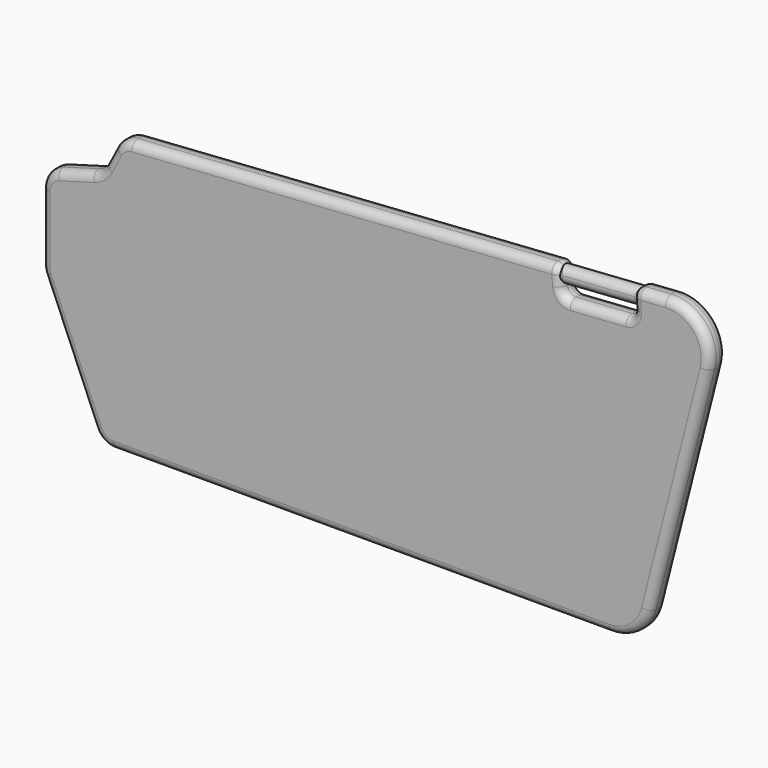
from build123d import *

# Parameters (mm, degrees)
F1_DEPTH      = 6.35
F2_R          = 12.7
F3_R          = 5.08
F5_DEPTH      = 50.8
F6_DEPTH      = 25.4
F7_T3_DEPTH   = 256.4039375074
F7_T6_DEPTH   = 256.4039375074
F7_T9_DEPTH   = 15.155251048
F7_T12_ANGLE  = 90
F7_S13_R      = 4.7625
F7_T14_DEPTH  = 6
F7_T17_ANGLE  = 108.2015581713
F7_T20_DEPTH  = 144.8369323212
F7_T23_ANGLE  = 90
F7_T26_ANGLE  = 75.7163995102
F7_T29_DEPTH  = 33.9682692967
F7_T32_DEPTH  = 302.1105912621
F7_T35_ANGLE  = 90
F7_T38_ANGLE  = 66.9516737984
F7_T41_DEPTH  = 78.7235310431
F7_T44_ANGLE  = 90
F7_S45_R      = 4.7625
F7_T46_DEPTH  = 6
F7_T49_ANGLE  = 23.0483262016
F7_T52_DEPTH  = 41.4021335168
F7_T55_ANGLE  = 58.5622729238
F7_T58_ANGLE  = 74.157776544
F7_T61_DEPTH  = 12.2118489341
F7_T64_DEPTH  = 22.3254991639
F7_T67_ANGLE  = 46.6380071493
F7_T70_DEPTH  = 15.155251048
F7_T73_ANGLE  = 90
F7_S74_R      = 4.7625
F7_T75_DEPTH  = 6
F7_T78_ANGLE  = 108.2015581713
F7_T81_DEPTH  = 144.8369323212
F7_T84_ANGLE  = 90
F7_T87_ANGLE  = 75.7163995102
F7_T90_DEPTH  = 33.9682692967
F7_T93_DEPTH  = 302.1105912621
F7_T96_ANGLE  = 90
F7_T99_ANGLE  = 66.9516737984
F7_T102_DEPTH = 78.7235310431
F7_T105_ANGLE = 90
F7_S106_R     = 4.7625
F7_T107_DEPTH = 6
F7_T110_ANGLE = 23.0483262016
F7_T113_DEPTH = 41.4021335168
F7_T116_ANGLE = 58.5622729238
F7_T119_ANGLE = 74.157776544
F7_T122_DEPTH = 12.2118489341
F7_T125_DEPTH = 22.3254991639
F7_T128_ANGLE = 46.6380071493
F7_T131_DEPTH = 6.35
F7_S132_R     = 4.7625
F7_T133_DEPTH = 7
F7_T136_DEPTH = 6.35
F7_S137_R     = 4.7625
F7_T138_DEPTH = 7
F7_T141_DEPTH = 6.35
F7_S142_R     = 4.7625
F7_T143_DEPTH = 7
F7_T146_DEPTH = 6.35
F7_S147_R     = 4.7625
F7_T148_DEPTH = 7


# Not quite as in the source:
# - a fillet or chamfer that OpenCascade refuses, or shapes differently, is made with other operations: its cross-section is extruded or revolved along the edge and cut away or added
# - a feature names something its author has since deleted; it is built from what else it names


with BuildPart() as f1:
    # F0 (on Front) → F1 (new body, symmetric)
    with BuildSketch(Plane.XZ):
        with BuildLine():
            Line((-207.3190157797, -14.1988740305), (-172.196418047, -96.7488740305))
            Line((-172.196418047, -96.7488740305), (138.3124196887, -96.7488740305))
            ThreePointArc((138.3124196887, -96.7488740305), (153.9006374043, -91.402987535), (162.9272139723, -77.6156038299))
            Line((162.9272139723, -77.6156038299), (198.6616202648, 62.7438959238))
            ThreePointArc((198.6616202648, 62.7438959238), (193.5563518445, 85.2752622268), (172.3112952336, 94.3512636991))
            Line((172.3112952336, 94.3512636991), (152.1233357391, 92.9686298258))
            Line((152.1233357391, 92.9686298258), (153.2514307251, 76.4972151415))
            Line((153.2514307251, 76.4972151415), (109.2262930579, 73.4820195428))
            Line((109.2262930579, 73.4820195428), (108.0981980719, 89.9534342271))
            Line((108.0981980719, 89.9534342271), (-159.8793958766, 71.6001727804))
            Line((-159.8793958766, 71.6001727804), (-171.3419263278, 49.5993942022))
            Line((-171.3419263278, 49.5993942022), (-207.3190157797, 39.3902622163))
            Line((-207.3190157797, 39.3902622163), (-207.3190157797, -14.1988740305))
        make_face()
    extrude(amount=F1_DEPTH, both=True)

    # F2
    f2_edges = [f1.edges().sort_by_distance(p)[0] for p in [
        (-171.341926, 0, 49.599394),
        (-207.319016, 0, 39.390262),
        (-159.879396, 0, 71.600173),
        (-207.319016, 0, -14.198874),
        (-172.196418, 0, -96.748874),
    ]]
    fillet(f2_edges, radius=F2_R)

    # F3
    f3_edges = [f1.edges().sort_by_distance(p)[0] for p in [
        (109.226293, 0, 73.48202),
        (153.251431, 0, 76.497215),
        (108.098198, 0, 89.953434),
        (152.123336, 0, 92.96863),
    ]]
    fillet(f3_edges, radius=F3_R)

    # F4 (on face) → F5 (join)
    with BuildSketch(Plane(origin=(113.7254907181, 0, 7.7888364977), x_dir=(0, 1, 0), z_dir=(0.9976629124, 0, 0.0683279822))):
        with BuildLine():
            Line((-4.686375775, 77.2770734216), (4.686375775, 77.2770734216))
            ThreePointArc((4.686375775, 77.2770734216), (0, 81.1914647341), (-4.686375775, 77.2770734216))
        make_face()
        with BuildLine():
            ThreePointArc((-4.686375775, 77.2770734216), (-0.4257590996, 71.6855339673), (4.7625, 76.4289647341))
            ThreePointArc((4.7625, 76.4289647341), (4.7434307668, 76.8547238336), (4.686375775, 77.2770734216))
            Line((4.686375775, 77.2770734216), (-4.686375775, 77.2770734216))
        make_face()
    extrude(amount=F5_DEPTH)

    # F6 (add): a face of the model
    f6_faces = [f1.faces().sort_by_distance(p)[0] for p in [
        (108.3333406106, 0, 86.5200972184),
    ]]
    extrude(f6_faces, amount=F6_DEPTH)

    # F7: fillet of radius 5.08 on 40 edges, made by hand


with BuildPart() as f7_tool1:
    # F7_s2 → F7_t3 (new body)
    with BuildSketch(Plane(origin=(108.657363123, 0, 7.4417303481), x_dir=(0, 1, 0), z_dir=(-0.9976629124, 0, -0.0683279822))):
        with BuildLine():
            ThreePointArc((-1.27, -82.3570734216), (-4.8621024484, -80.86917587), (-6.35, -77.2770734216))
            Line((-6.35, -77.2770734216), (-6.35, -82.3570734216))
            Line((-6.35, -82.3570734216), (-1.27, -82.3570734216))
        make_face()
    extrude(amount=F7_T3_DEPTH)


with BuildPart() as f7_tool4:
    # F7_s5 → F7_t6 (new body)
    with BuildSketch(Plane(origin=(108.657363123, 0, 7.4417303481), x_dir=(0, 1, 0), z_dir=(-0.9976629124, 0, -0.0683279822))):
        with BuildLine():
            ThreePointArc((6.35, -77.2770734216), (4.8621024484, -80.86917587), (1.27, -82.3570734216))
            Line((1.27, -82.3570734216), (6.35, -82.3570734216))
            Line((6.35, -82.3570734216), (6.35, -77.2770734216))
        make_face()
    extrude(amount=F7_T6_DEPTH)


with BuildPart() as f7_tool7:
    # F7_s8 → F7_t9 (new body)
    with BuildSketch(Plane(origin=(177.9385878798, 0, 12.1866659697), x_dir=(0, 1, 0), z_dir=(-0.9976629124, 0, -0.0683279822))):
        with BuildLine():
            ThreePointArc((6.35, -77.2770734216), (4.8621024484, -80.86917587), (1.27, -82.3570734216))
            Line((1.27, -82.3570734216), (6.35, -82.3570734216))
            Line((6.35, -82.3570734216), (6.35, -77.2770734216))
        make_face()
    extrude(amount=F7_T9_DEPTH)


with BuildPart() as f7_tool10:
    # F7_s11 → F7_t12 (revolve)
    with BuildSketch(Plane(origin=(162.8187559806, 0, 11.1511382459), x_dir=(0, 1, 0), z_dir=(0.9976629124, 0, 0.0683279822))):
        with BuildLine():
            ThreePointArc((6.35, 77.2770734216), (4.8621024484, 80.86917587), (1.27, 82.3570734216))
            Line((1.27, 82.3570734216), (6.35, 82.3570734216))
            Line((6.35, 82.3570734216), (6.35, 77.2770734216))
        make_face()
    revolve(axis=Axis((157.5385694838, 6.35, 88.2476083802), (0, -1, 0)), revolution_arc=F7_T12_ANGLE)

    # F7_s13 → F7_t14 (cut, symmetric)
    with BuildSketch(Plane(origin=(160.4241963196, 0, 10.9871395367), x_dir=(0, 1, 0), z_dir=(-0.9976629124, 0, -0.0683279822))):
        with Locations((0, -76.4289647341)):
            Circle(F7_S13_R)
    extrude(amount=F7_T14_DEPTH, both=True, mode=Mode.SUBTRACT)


with BuildPart() as f7_tool15:
    # F7_s16 → F7_t17 (revolve)
    with BuildSketch(Plane(origin=(27.0945707988, 0, 106.4234948309), x_dir=(0, 1, 0), z_dir=(-0.2467216456, 0, -0.9690863891))):
        with BuildLine():
            ThreePointArc((6.35, 171.9599949818), (4.8621024484, 175.5520974303), (1.27, 177.0399949818))
            Line((1.27, 177.0399949818), (6.35, 177.0399949818))
            Line((6.35, 177.0399949818), (6.35, 171.9599949818))
        make_face()
    revolve(axis=Axis((174.0468259813, 6.35, 69.0106257232), (0, -1, 0)), revolution_arc=F7_T17_ANGLE)


with BuildPart() as f7_tool18:
    # F7_s19 → F7_t20 (new body)
    with BuildSketch(Plane(origin=(-8.6398354938, 0, -33.9360049229), x_dir=(0, 1, 0), z_dir=(0.2467216456, 0, 0.9690863891))):
        with BuildLine():
            ThreePointArc((6.35, -171.9599949818), (4.8621024484, -175.5520974303), (1.27, -177.0399949818))
            Line((1.27, -177.0399949818), (6.35, -177.0399949818))
            Line((6.35, -177.0399949818), (6.35, -171.9599949818))
        make_face()
    extrude(amount=F7_T20_DEPTH)


with BuildPart() as f7_tool21:
    # F7_s22 → F7_t23 (revolve)
    with BuildSketch(Plane(origin=(-4.8463038098, 0, 70.7613106403), x_dir=(0, 1, 0), z_dir=(-0.0683279822, 0, 0.9976629124))):
        with BuildLine():
            ThreePointArc((6.35, -163.2001690662), (4.8621024484, -159.6080666178), (1.27, -158.1201690662))
            Line((1.27, -158.1201690662), (6.35, -158.1201690662))
            Line((6.35, -158.1201690662), (6.35, -163.2001690662))
        make_face()
    revolve(axis=Axis((147.8361969804, 6.35, 81.2182365871), (0, 1, 0)), revolution_arc=F7_T23_ANGLE)


with BuildPart() as f7_tool24:
    # F7_s25 → F7_t26 (revolve)
    with BuildSketch(Plane.YZ.offset(138.3124196887)):
        with BuildLine():
            ThreePointArc((6.35, -91.6688740305), (4.8621024484, -95.2609764789), (1.27, -96.7488740305))
            Line((1.27, -96.7488740305), (6.35, -96.7488740305))
            Line((6.35, -96.7488740305), (6.35, -91.6688740305))
        make_face()
    revolve(axis=Axis((138.3124196887, 6.35, -71.3488740305), (0, -1, 0)), revolution_arc=F7_T26_ANGLE)


with BuildPart() as f7_tool27:
    # F7_s28 → F7_t29 (new body)
    with BuildSketch(Plane(origin=(152.6825007902, 0, 10.4569259469), x_dir=(0, 1, 0), z_dir=(-0.9976629124, 0, -0.0683279822))):
        with BuildLine():
            ThreePointArc((6.35, -60.7670734216), (4.8621024484, -64.35917587), (1.27, -65.8470734216))
            Line((1.27, -65.8470734216), (6.35, -65.8470734216))
            Line((6.35, -65.8470734216), (6.35, -60.7670734216))
        make_face()
    extrude(amount=F7_T29_DEPTH)


with BuildPart() as f7_tool30:
    # F7_s31 → F7_t32 (new body)
    with BuildSketch(Plane.YZ.offset(-163.7981715734)):
        with BuildLine():
            ThreePointArc((6.35, -91.6688740305), (4.8621024484, -95.2609764789), (1.27, -96.7488740305))
            Line((1.27, -96.7488740305), (6.35, -96.7488740305))
            Line((6.35, -96.7488740305), (6.35, -91.6688740305))
        make_face()
    extrude(amount=F7_T32_DEPTH)


with BuildPart() as f7_tool33:
    # F7_s34 → F7_t35 (revolve)
    with BuildSketch(Plane(origin=(118.7936183133, 0, 8.1359426472), x_dir=(0, 1, 0), z_dir=(0.9976629124, 0, 0.0683279822))):
        with BuildLine():
            ThreePointArc((6.35, 60.7670734216), (4.8621024484, 64.35917587), (1.27, 65.8470734216))
            Line((1.27, 65.8470734216), (6.35, 65.8470734216))
            Line((6.35, 65.8470734216), (6.35, 60.7670734216))
        make_face()
    revolve(axis=Axis((113.9473145035, 6.35, 78.8972532875), (0, 1, 0)), revolution_arc=F7_T35_ANGLE)


with BuildPart() as f7_tool36:
    # F7_s37 → F7_t38 (revolve)
    with BuildSketch(Plane(origin=(5.1723900497, 0, -12.1568684029), x_dir=(0, 1, 0), z_dir=(-0.3915073905, 0, 0.9201749634))):
        with BuildLine():
            ThreePointArc((6.35, 191.2487318706), (4.8621024484, 194.840834319), (1.27, 196.3287318706))
            Line((1.27, 196.3287318706), (6.35, 196.3287318706))
            Line((6.35, 196.3287318706), (6.35, 191.2487318706))
        make_face()
    revolve(axis=Axis((-163.7981715734, 6.35, -84.0488740305), (0, -1, 0)), revolution_arc=F7_T38_ANGLE)


with BuildPart() as f7_tool39:
    # F7_s40 → F7_t41 (new body)
    with BuildSketch(Plane(origin=(-25.6484541565, 0, 60.2825538912), x_dir=(0, 1, 0), z_dir=(0.3915073905, 0, -0.9201749634))):
        with BuildLine():
            ThreePointArc((6.35, -191.2487318706), (4.8621024484, -194.840834319), (1.27, -196.3287318706))
            Line((1.27, -196.3287318706), (6.35, -196.3287318706))
            Line((6.35, -196.3287318706), (6.35, -191.2487318706))
        make_face()
    extrude(amount=F7_T41_DEPTH)


with BuildPart() as f7_tool42:
    # F7_s43 → F7_t44 (revolve)
    with BuildSketch(Plane(origin=(108.657363123, 0, 7.4417303481), x_dir=(0, 1, 0), z_dir=(-0.9976629124, 0, -0.0683279822))):
        with BuildLine():
            ThreePointArc((6.35, -77.2770734216), (4.8621024484, -80.86917587), (1.27, -82.3570734216))
            Line((1.27, -82.3570734216), (6.35, -82.3570734216))
            Line((6.35, -82.3570734216), (6.35, -77.2770734216))
        make_face()
    revolve(axis=Axis((103.3771766262, 6.35, 84.5382004824), (0, 1, 0)), revolution_arc=F7_T44_ANGLE)

    # F7_s45 → F7_t46 (cut, symmetric)
    with BuildSketch(Plane(origin=(111.1396484453, 0, 7.6117372164), x_dir=(0, 1, 0), z_dir=(-0.9976629124, 0, -0.0683279822))):
        with Locations((0, -76.4289647341)):
            Circle(F7_S45_R)
    extrude(amount=F7_T46_DEPTH, both=True, mode=Mode.SUBTRACT)


with BuildPart() as f7_tool47:
    # F7_s48 → F7_t49 (revolve)
    with BuildSketch(Plane(origin=(-25.6484541565, 0, 60.2825538912), x_dir=(0, 1, 0), z_dir=(0.3915073905, 0, -0.9201749634))):
        with BuildLine():
            ThreePointArc((6.35, -191.2487318706), (4.8621024484, -194.840834319), (1.27, -196.3287318706))
            Line((1.27, -196.3287318706), (6.35, -196.3287318706))
            Line((6.35, -196.3287318706), (6.35, -191.2487318706))
        make_face()
    revolve(axis=Axis((-194.6190157797, 6.35, -11.6094517364), (0, 1, 0)), revolution_arc=F7_T49_ANGLE)


with BuildPart() as f7_tool50:
    # F7_s51 → F7_t52 (new body)
    with BuildSketch(Plane.XY.offset(29.7926817804)):
        with BuildLine():
            ThreePointArc((-202.2390157797, 6.35), (-205.8311182281, 4.8621024484), (-207.3190157797, 1.27))
            Line((-207.3190157797, 1.27), (-207.3190157797, 6.35))
            Line((-207.3190157797, 6.35), (-202.2390157797, 6.35))
        make_face()
    extrude(amount=-F7_T52_DEPTH)


with BuildPart() as f7_tool53:
    # F7_s54 → F7_t55 (revolve)
    with BuildSketch(Plane(origin=(-8.0839739406, 0, -15.5160958095), x_dir=(0, 1, 0), z_dir=(-0.4620546409, 0, -0.8868514582))):
        with BuildLine():
            ThreePointArc((6.35, -169.7924674841), (4.8621024484, -173.3845699325), (1.27, -174.8724674841))
            Line((1.27, -174.8724674841), (6.35, -174.8724674841))
            Line((6.35, -174.8724674841), (6.35, -169.7924674841))
        make_face()
    revolve(axis=Axis((-151.906863203, 6.35, 59.4164454132), (0, 1, 0)), revolution_arc=F7_T55_ANGLE)


with BuildPart() as f7_tool56:
    # F7_s57 → F7_t58 (revolve)
    with BuildSketch(Plane.XY.offset(29.7926817804)):
        with BuildLine():
            ThreePointArc((-202.2390157797, 6.35), (-205.8311182281, 4.8621024484), (-207.3190157797, 1.27))
            Line((-207.3190157797, 1.27), (-207.3190157797, 6.35))
            Line((-207.3190157797, 6.35), (-202.2390157797, 6.35))
        make_face()
    revolve(axis=Axis((-194.6190157797, 6.35, 29.7926817804), (0, 1, 0)), revolution_arc=F7_T58_ANGLE)


with BuildPart() as f7_tool59:
    # F7_s60 → F7_t61 (new body)
    with BuildSketch(Plane(origin=(-8.0839739406, 0, -15.5160958095), x_dir=(0, 1, 0), z_dir=(-0.4620546409, 0, -0.8868514582))):
        with BuildLine():
            ThreePointArc((6.35, -169.7924674841), (4.8621024484, -173.3845699325), (1.27, -174.8724674841))
            Line((1.27, -174.8724674841), (6.35, -174.8724674841))
            Line((6.35, -174.8724674841), (6.35, -169.7924674841))
        make_face()
    extrude(amount=F7_T61_DEPTH)


with BuildPart() as f7_tool62:
    # F7_s63 → F7_t64 (new body)
    with BuildSketch(Plane(origin=(-150.8137198417, 0, -42.7960458894), x_dir=(0, 1, 0), z_dir=(-0.9620170785, 0, -0.2729892684))):
        with BuildLine():
            ThreePointArc((6.35, -89.4099714147), (4.8621024484, -93.0020738631), (1.27, -94.4899714147))
            Line((1.27, -94.4899714147), (6.35, -94.4899714147))
            Line((6.35, -94.4899714147), (6.35, -89.4099714147))
        make_face()
    extrude(amount=F7_T64_DEPTH)


with BuildPart() as f7_tool65:
    # F7_s66 → F7_t67 (revolve)
    with BuildSketch(Plane(origin=(-150.8137198417, 0, -42.7960458894), x_dir=(0, 1, 0), z_dir=(-0.9620170785, 0, -0.2729892684))):
        with BuildLine():
            ThreePointArc((6.35, -89.4099714147), (4.8621024484, -93.0020738631), (1.27, -94.4899714147))
            Line((1.27, -94.4899714147), (6.35, -94.4899714147))
            Line((6.35, -94.4899714147), (6.35, -89.4099714147))
        make_face()
    revolve(axis=Axis((-180.075431714, 6.35, 60.3225372573), (0, -1, 0)), revolution_arc=F7_T67_ANGLE)


with BuildPart() as f7_tool68:
    # F7_s69 → F7_t70 (new body)
    with BuildSketch(Plane(origin=(177.9385878798, 0, 12.1866659697), x_dir=(0, 1, 0), z_dir=(-0.9976629124, 0, -0.0683279822))):
        with BuildLine():
            ThreePointArc((-1.27, -82.3570734216), (-4.8621024484, -80.86917587), (-6.35, -77.2770734216))
            Line((-6.35, -77.2770734216), (-6.35, -82.3570734216))
            Line((-6.35, -82.3570734216), (-1.27, -82.3570734216))
        make_face()
    extrude(amount=F7_T70_DEPTH)


with BuildPart() as f7_tool71:
    # F7_s72 → F7_t73 (revolve)
    with BuildSketch(Plane(origin=(162.8187559806, 0, 11.1511382459), x_dir=(0, 1, 0), z_dir=(0.9976629124, 0, 0.0683279822))):
        with BuildLine():
            ThreePointArc((-1.27, 82.3570734216), (-4.8621024484, 80.86917587), (-6.35, 77.2770734216))
            Line((-6.35, 77.2770734216), (-6.35, 82.3570734216))
            Line((-6.35, 82.3570734216), (-1.27, 82.3570734216))
        make_face()
    revolve(axis=Axis((157.5385694838, -6.35, 88.2476083802), (0, -1, 0)), revolution_arc=F7_T73_ANGLE)

    # F7_s74 → F7_t75 (cut, symmetric)
    with BuildSketch(Plane(origin=(160.4241963196, 0, 10.9871395367), x_dir=(0, 1, 0), z_dir=(-0.9976629124, 0, -0.0683279822))):
        with Locations((0, -76.4289647341)):
            Circle(F7_S74_R)
    extrude(amount=F7_T75_DEPTH, both=True, mode=Mode.SUBTRACT)


with BuildPart() as f7_tool76:
    # F7_s77 → F7_t78 (revolve)
    with BuildSketch(Plane(origin=(27.0945707988, 0, 106.4234948309), x_dir=(0, 1, 0), z_dir=(-0.2467216456, 0, -0.9690863891))):
        with BuildLine():
            ThreePointArc((-1.27, 177.0399949818), (-4.8621024484, 175.5520974303), (-6.35, 171.9599949818))
            Line((-6.35, 171.9599949818), (-6.35, 177.0399949818))
            Line((-6.35, 177.0399949818), (-1.27, 177.0399949818))
        make_face()
    revolve(axis=Axis((174.0468259813, -6.35, 69.0106257232), (0, -1, 0)), revolution_arc=F7_T78_ANGLE)


with BuildPart() as f7_tool79:
    # F7_s80 → F7_t81 (new body)
    with BuildSketch(Plane(origin=(-8.6398354938, 0, -33.9360049229), x_dir=(0, 1, 0), z_dir=(0.2467216456, 0, 0.9690863891))):
        with BuildLine():
            ThreePointArc((-1.27, -177.0399949818), (-4.8621024484, -175.5520974303), (-6.35, -171.9599949818))
            Line((-6.35, -171.9599949818), (-6.35, -177.0399949818))
            Line((-6.35, -177.0399949818), (-1.27, -177.0399949818))
        make_face()
    extrude(amount=F7_T81_DEPTH)


with BuildPart() as f7_tool82:
    # F7_s83 → F7_t84 (revolve)
    with BuildSketch(Plane(origin=(-4.8463038098, 0, 70.7613106403), x_dir=(0, 1, 0), z_dir=(-0.0683279822, 0, 0.9976629124))):
        with BuildLine():
            ThreePointArc((-1.27, -158.1201690662), (-4.8621024484, -159.6080666178), (-6.35, -163.2001690662))
            Line((-6.35, -163.2001690662), (-6.35, -158.1201690662))
            Line((-6.35, -158.1201690662), (-1.27, -158.1201690662))
        make_face()
    revolve(axis=Axis((147.8361969804, -6.35, 81.2182365871), (0, 1, 0)), revolution_arc=F7_T84_ANGLE)


with BuildPart() as f7_tool85:
    # F7_s86 → F7_t87 (revolve)
    with BuildSketch(Plane.YZ.offset(138.3124196887)):
        with BuildLine():
            ThreePointArc((-1.27, -96.7488740305), (-4.8621024484, -95.2609764789), (-6.35, -91.6688740305))
            Line((-6.35, -91.6688740305), (-6.35, -96.7488740305))
            Line((-6.35, -96.7488740305), (-1.27, -96.7488740305))
        make_face()
    revolve(axis=Axis((138.3124196887, -6.35, -71.3488740305), (0, -1, 0)), revolution_arc=F7_T87_ANGLE)


with BuildPart() as f7_tool88:
    # F7_s89 → F7_t90 (new body)
    with BuildSketch(Plane(origin=(152.6825007902, 0, 10.4569259469), x_dir=(0, 1, 0), z_dir=(-0.9976629124, 0, -0.0683279822))):
        with BuildLine():
            ThreePointArc((-1.27, -65.8470734216), (-4.8621024484, -64.35917587), (-6.35, -60.7670734216))
            Line((-6.35, -60.7670734216), (-6.35, -65.8470734216))
            Line((-6.35, -65.8470734216), (-1.27, -65.8470734216))
        make_face()
    extrude(amount=F7_T90_DEPTH)


with BuildPart() as f7_tool91:
    # F7_s92 → F7_t93 (new body)
    with BuildSketch(Plane.YZ.offset(-163.7981715734)):
        with BuildLine():
            ThreePointArc((-1.27, -96.7488740305), (-4.8621024484, -95.2609764789), (-6.35, -91.6688740305))
            Line((-6.35, -91.6688740305), (-6.35, -96.7488740305))
            Line((-6.35, -96.7488740305), (-1.27, -96.7488740305))
        make_face()
    extrude(amount=F7_T93_DEPTH)


with BuildPart() as f7_tool94:
    # F7_s95 → F7_t96 (revolve)
    with BuildSketch(Plane(origin=(118.7936183133, 0, 8.1359426472), x_dir=(0, 1, 0), z_dir=(0.9976629124, 0, 0.0683279822))):
        with BuildLine():
            ThreePointArc((-1.27, 65.8470734216), (-4.8621024484, 64.35917587), (-6.35, 60.7670734216))
            Line((-6.35, 60.7670734216), (-6.35, 65.8470734216))
            Line((-6.35, 65.8470734216), (-1.27, 65.8470734216))
        make_face()
    revolve(axis=Axis((113.9473145035, -6.35, 78.8972532875), (0, 1, 0)), revolution_arc=F7_T96_ANGLE)


with BuildPart() as f7_tool97:
    # F7_s98 → F7_t99 (revolve)
    with BuildSketch(Plane(origin=(5.1723900497, 0, -12.1568684029), x_dir=(0, 1, 0), z_dir=(-0.3915073905, 0, 0.9201749634))):
        with BuildLine():
            ThreePointArc((-1.27, 196.3287318706), (-4.8621024484, 194.840834319), (-6.35, 191.2487318706))
            Line((-6.35, 191.2487318706), (-6.35, 196.3287318706))
            Line((-6.35, 196.3287318706), (-1.27, 196.3287318706))
        make_face()
    revolve(axis=Axis((-163.7981715734, -6.35, -84.0488740305), (0, -1, 0)), revolution_arc=F7_T99_ANGLE)


with BuildPart() as f7_tool100:
    # F7_s101 → F7_t102 (new body)
    with BuildSketch(Plane(origin=(-25.6484541565, 0, 60.2825538912), x_dir=(0, 1, 0), z_dir=(0.3915073905, 0, -0.9201749634))):
        with BuildLine():
            ThreePointArc((-1.27, -196.3287318706), (-4.8621024484, -194.840834319), (-6.35, -191.2487318706))
            Line((-6.35, -191.2487318706), (-6.35, -196.3287318706))
            Line((-6.35, -196.3287318706), (-1.27, -196.3287318706))
        make_face()
    extrude(amount=F7_T102_DEPTH)


with BuildPart() as f7_tool103:
    # F7_s104 → F7_t105 (revolve)
    with BuildSketch(Plane(origin=(108.657363123, 0, 7.4417303481), x_dir=(0, 1, 0), z_dir=(-0.9976629124, 0, -0.0683279822))):
        with BuildLine():
            ThreePointArc((-1.27, -82.3570734216), (-4.8621024484, -80.86917587), (-6.35, -77.2770734216))
            Line((-6.35, -77.2770734216), (-6.35, -82.3570734216))
            Line((-6.35, -82.3570734216), (-1.27, -82.3570734216))
        make_face()
    revolve(axis=Axis((103.3771766262, -6.35, 84.5382004824), (0, 1, 0)), revolution_arc=F7_T105_ANGLE)

    # F7_s106 → F7_t107 (cut, symmetric)
    with BuildSketch(Plane(origin=(111.1396484453, 0, 7.6117372164), x_dir=(0, 1, 0), z_dir=(-0.9976629124, 0, -0.0683279822))):
        with Locations((0, -76.4289647341)):
            Circle(F7_S106_R)
    extrude(amount=F7_T107_DEPTH, both=True, mode=Mode.SUBTRACT)


with BuildPart() as f7_tool108:
    # F7_s109 → F7_t110 (revolve)
    with BuildSketch(Plane(origin=(-25.6484541565, 0, 60.2825538912), x_dir=(0, 1, 0), z_dir=(0.3915073905, 0, -0.9201749634))):
        with BuildLine():
            ThreePointArc((-1.27, -196.3287318706), (-4.8621024484, -194.840834319), (-6.35, -191.2487318706))
            Line((-6.35, -191.2487318706), (-6.35, -196.3287318706))
            Line((-6.35, -196.3287318706), (-1.27, -196.3287318706))
        make_face()
    revolve(axis=Axis((-194.6190157797, -6.35, -11.6094517364), (0, 1, 0)), revolution_arc=F7_T110_ANGLE)


with BuildPart() as f7_tool111:
    # F7_s112 → F7_t113 (new body)
    with BuildSketch(Plane.XY.offset(29.7926817804)):
        with BuildLine():
            ThreePointArc((-207.3190157797, -1.27), (-205.8311182281, -4.8621024484), (-202.2390157797, -6.35))
            Line((-202.2390157797, -6.35), (-207.3190157797, -6.35))
            Line((-207.3190157797, -6.35), (-207.3190157797, -1.27))
        make_face()
    extrude(amount=-F7_T113_DEPTH)


with BuildPart() as f7_tool114:
    # F7_s115 → F7_t116 (revolve)
    with BuildSketch(Plane(origin=(-8.0839739406, 0, -15.5160958095), x_dir=(0, 1, 0), z_dir=(-0.4620546409, 0, -0.8868514582))):
        with BuildLine():
            ThreePointArc((-1.27, -174.8724674841), (-4.8621024484, -173.3845699325), (-6.35, -169.7924674841))
            Line((-6.35, -169.7924674841), (-6.35, -174.8724674841))
            Line((-6.35, -174.8724674841), (-1.27, -174.8724674841))
        make_face()
    revolve(axis=Axis((-151.906863203, -6.35, 59.4164454132), (0, 1, 0)), revolution_arc=F7_T116_ANGLE)


with BuildPart() as f7_tool117:
    # F7_s118 → F7_t119 (revolve)
    with BuildSketch(Plane.XY.offset(29.7926817804)):
        with BuildLine():
            ThreePointArc((-207.3190157797, -1.27), (-205.8311182281, -4.8621024484), (-202.2390157797, -6.35))
            Line((-202.2390157797, -6.35), (-207.3190157797, -6.35))
            Line((-207.3190157797, -6.35), (-207.3190157797, -1.27))
        make_face()
    revolve(axis=Axis((-194.6190157797, -6.35, 29.7926817804), (0, 1, 0)), revolution_arc=F7_T119_ANGLE)


with BuildPart() as f7_tool120:
    # F7_s121 → F7_t122 (new body)
    with BuildSketch(Plane(origin=(-8.0839739406, 0, -15.5160958095), x_dir=(0, 1, 0), z_dir=(-0.4620546409, 0, -0.8868514582))):
        with BuildLine():
            ThreePointArc((-1.27, -174.8724674841), (-4.8621024484, -173.3845699325), (-6.35, -169.7924674841))
            Line((-6.35, -169.7924674841), (-6.35, -174.8724674841))
            Line((-6.35, -174.8724674841), (-1.27, -174.8724674841))
        make_face()
    extrude(amount=F7_T122_DEPTH)


with BuildPart() as f7_tool123:
    # F7_s124 → F7_t125 (new body)
    with BuildSketch(Plane(origin=(-150.8137198417, 0, -42.7960458894), x_dir=(0, 1, 0), z_dir=(-0.9620170785, 0, -0.2729892684))):
        with BuildLine():
            ThreePointArc((-1.27, -94.4899714147), (-4.8621024484, -93.0020738631), (-6.35, -89.4099714147))
            Line((-6.35, -89.4099714147), (-6.35, -94.4899714147))
            Line((-6.35, -94.4899714147), (-1.27, -94.4899714147))
        make_face()
    extrude(amount=F7_T125_DEPTH)


with BuildPart() as f7_tool126:
    # F7_s127 → F7_t128 (revolve)
    with BuildSketch(Plane(origin=(-150.8137198417, 0, -42.7960458894), x_dir=(0, 1, 0), z_dir=(-0.9620170785, 0, -0.2729892684))):
        with BuildLine():
            ThreePointArc((-1.27, -94.4899714147), (-4.8621024484, -93.0020738631), (-6.35, -89.4099714147))
            Line((-6.35, -89.4099714147), (-6.35, -94.4899714147))
            Line((-6.35, -94.4899714147), (-1.27, -94.4899714147))
        make_face()
    revolve(axis=Axis((-180.075431714, -6.35, 60.3225372573), (0, -1, 0)), revolution_arc=F7_T128_ANGLE)


with BuildPart() as f7_tool129:
    # F7_s130 → F7_t131 (new body)
    with BuildSketch(Plane(origin=(-4.8463038098, 0, 70.7613106403), x_dir=(0, 1, 0), z_dir=(-0.0683279822, 0, 0.9976629124))):
        with BuildLine():
            ThreePointArc((-1.27, -113.9918997695), (-4.8621024484, -112.504002218), (-6.35, -108.9118997695))
            Line((-6.35, -108.9118997695), (-6.35, -113.9918997695))
            Line((-6.35, -113.9918997695), (-1.27, -113.9918997695))
        make_face()
    extrude(amount=F7_T131_DEPTH)

    # F7_s132 → F7_t133 (cut, symmetric)
    with BuildSketch(Plane(origin=(111.2394147366, 0, 7.6185700146), x_dir=(0, 1, 0), z_dir=(-0.9976629124, 0, -0.0683279822))):
        with Locations((0, -76.4289647341)):
            Circle(F7_S132_R)
    extrude(amount=F7_T133_DEPTH, both=True, mode=Mode.SUBTRACT)


with BuildPart() as f7_tool134:
    # F7_s135 → F7_t136 (new body)
    with BuildSketch(Plane(origin=(-5.2801864967, 0, 77.0964701342), x_dir=(0, 1, 0), z_dir=(0.0683279822, 0, -0.9976629124))):
        with BuildLine():
            ThreePointArc((-1.27, 158.1201690662), (-4.8621024484, 159.6080666178), (-6.35, 163.2001690662))
            Line((-6.35, 163.2001690662), (-6.35, 158.1201690662))
            Line((-6.35, 158.1201690662), (-1.27, 158.1201690662))
        make_face()
    extrude(amount=F7_T136_DEPTH)

    # F7_s137 → F7_t138 (cut, symmetric)
    with BuildSketch(Plane(origin=(160.3244300284, 0, 10.9803067385), x_dir=(0, 1, 0), z_dir=(-0.9976629124, 0, -0.0683279822))):
        with Locations((0, -76.4289647341)):
            Circle(F7_S137_R)
    extrude(amount=F7_T138_DEPTH, both=True, mode=Mode.SUBTRACT)


with BuildPart() as f7_tool139:
    # F7_s140 → F7_t141 (new body)
    with BuildSketch(Plane(origin=(-4.8463038098, 0, 70.7613106403), x_dir=(0, 1, 0), z_dir=(-0.0683279822, 0, 0.9976629124))):
        with BuildLine():
            ThreePointArc((6.35, -108.9118997695), (4.8621024484, -112.504002218), (1.27, -113.9918997695))
            Line((1.27, -113.9918997695), (6.35, -113.9918997695))
            Line((6.35, -113.9918997695), (6.35, -108.9118997695))
        make_face()
    extrude(amount=F7_T141_DEPTH)

    # F7_s142 → F7_t143 (cut, symmetric)
    with BuildSketch(Plane(origin=(111.2394147366, 0, 7.6185700146), x_dir=(0, 1, 0), z_dir=(-0.9976629124, 0, -0.0683279822))):
        with Locations((0, -76.4289647341)):
            Circle(F7_S142_R)
    extrude(amount=F7_T143_DEPTH, both=True, mode=Mode.SUBTRACT)


with BuildPart() as f7_tool144:
    # F7_s145 → F7_t146 (new body)
    with BuildSketch(Plane(origin=(-5.2801864967, 0, 77.0964701342), x_dir=(0, 1, 0), z_dir=(0.0683279822, 0, -0.9976629124))):
        with BuildLine():
            ThreePointArc((6.35, 163.2001690662), (4.8621024484, 159.6080666178), (1.27, 158.1201690662))
            Line((1.27, 158.1201690662), (6.35, 158.1201690662))
            Line((6.35, 158.1201690662), (6.35, 163.2001690662))
        make_face()
    extrude(amount=F7_T146_DEPTH)

    # F7_s147 → F7_t148 (cut, symmetric)
    with BuildSketch(Plane(origin=(160.3244300284, 0, 10.9803067385), x_dir=(0, 1, 0), z_dir=(-0.9976629124, 0, -0.0683279822))):
        with Locations((0, -76.4289647341)):
            Circle(F7_S147_R)
    extrude(amount=F7_T148_DEPTH, both=True, mode=Mode.SUBTRACT)


with BuildPart() as f1_1:
    add(f1.part)

    # F7_t149: cut F7_tool1, F7_tool4, F7_tool7, F7_tool10, F7_tool15, F7_tool18, F7_tool21, F7_tool24, F7_tool27, F7_tool30, F7_tool33, F7_tool36, F7_tool39, F7_tool42, F7_tool47, F7_tool50, F7_tool53, F7_tool56, F7_tool59, F7_tool62, F7_tool65, F7_tool68, F7_tool71, F7_tool76, F7_tool79, F7_tool82, F7_tool85, F7_tool88, F7_tool91, F7_tool94, F7_tool97, F7_tool100, F7_tool103, F7_tool108, F7_tool111, F7_tool114, F7_tool117, F7_tool120, F7_tool123, F7_tool126, F7_tool129, F7_tool134, F7_tool139, F7_tool144
    add([f7_tool1.part, f7_tool4.part, f7_tool7.part, f7_tool10.part, f7_tool15.part, f7_tool18.part, f7_tool21.part, f7_tool24.part, f7_tool27.part, f7_tool30.part, f7_tool33.part, f7_tool36.part, f7_tool39.part, f7_tool42.part, f7_tool47.part, f7_tool50.part, f7_tool53.part, f7_tool56.part, f7_tool59.part, f7_tool62.part, f7_tool65.part, f7_tool68.part, f7_tool71.part, f7_tool76.part, f7_tool79.part, f7_tool82.part, f7_tool85.part, f7_tool88.part, f7_tool91.part, f7_tool94.part, f7_tool97.part, f7_tool100.part, f7_tool103.part, f7_tool108.part, f7_tool111.part, f7_tool114.part, f7_tool117.part, f7_tool120.part, f7_tool123.part, f7_tool126.part, f7_tool129.part, f7_tool134.part, f7_tool139.part, f7_tool144.part], mode=Mode.SUBTRACT)


solid = f1_1.part
